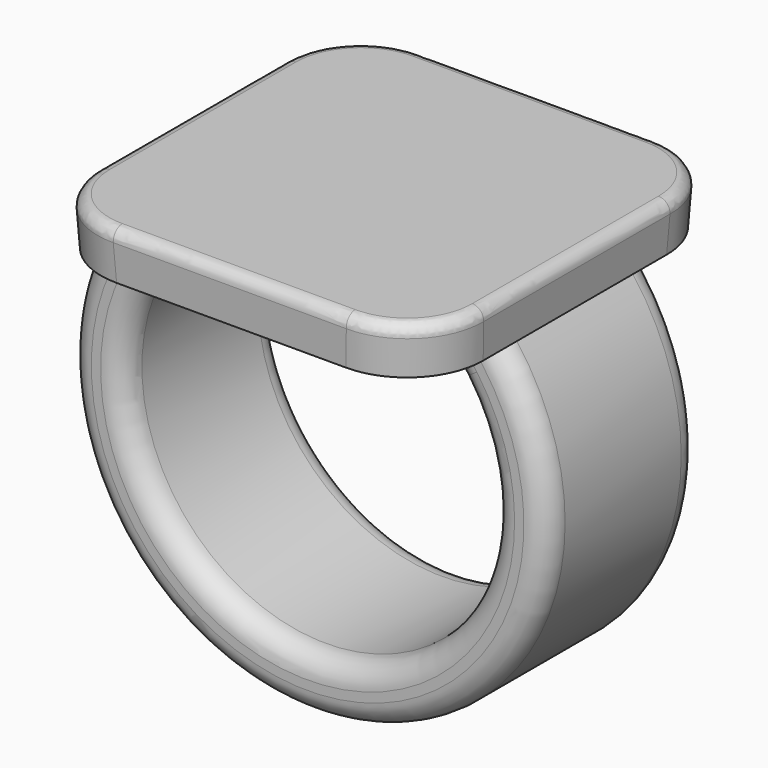
from build123d import *

# Parameters (mm, degrees)
F0_W          = 25.4
F0_H          = 25.4
F1_DEPTH      = 3.175
F1_TAPER      = -3
F3_W          = 5.08
F3_H          = 12.7
F6_DEPTH      = 6.35
F6_DEPTH_BACK = 6.35
F7_R          = 5.08
F8_R          = 1.524
F9_R          = 0.762


# Not quite as in the source:
# - a feature names something its author has since deleted; it is built from what else it names


with BuildPart() as f1:
    # F0 (on Top) → F1 (new body)
    with BuildSketch(Plane.XY):
        Rectangle(F0_W, F0_H)
    extrude(amount=F1_DEPTH, taper=F1_TAPER)

    # F4: sweep along a path in F2
    with BuildLine(Plane.XZ) as f4_path:
        ThreePointArc((-10.16, 0), (0, -23.5582897328), (10.16, 0))
    # F3 (on face) → F4 (sweep)
    with BuildSketch(Plane(origin=(0, 0, 0), x_dir=(1, 0, 0), z_dir=(0, 0, -1))):
        with Locations((-10.16, 0)):
            Rectangle(F3_W, F3_H)
    sweep(path=f4_path.line)

    # F5 (on Front) → F6 (join, two sides)
    with BuildSketch(Plane.XZ) as f6_sk:
        with BuildLine():
            Line((10.0130578512, -2.535746045), (10.16, 0))
            Line((10.16, 0), (7.62, 0))
            ThreePointArc((7.62, 0), (8.9072265211, -1.1822790439), (10.0130578512, -2.535746045))
        make_face()
    extrude(amount=F6_DEPTH)
    extrude(f6_sk.sketch, amount=-F6_DEPTH_BACK)

    # F7
    f7_edges = [f1.edges().sort_by_distance(p)[0] for p in [
        (-12.783197, 12.783197, 1.5875),
        (-12.783197, -12.783197, 1.5875),
        (12.783197, -12.783197, 1.5875),
        (12.783197, 12.783197, 1.5875),
    ]]
    fillet(f7_edges, radius=F7_R)

    # F8
    f8_edges = [f1.edges().sort_by_distance(p)[0] for p in [
        (-1.743325, -6.35, -21.711017),
        (8.907227, -6.35, -1.182279),
        (-1.743325, 6.35, -21.711017),
        (0, -6.35, -25.501344),
        (8.907227, 6.35, -1.182279),
        (0, 6.35, -25.501344),
    ]]
    fillet(f8_edges, radius=F8_R)

    # F9
    f9_edges = [f1.edges().sort_by_distance(p)[0] for p in [
        (0, -12.866395, 3.175),
        (-11.381378, -11.381378, 3.175),
        (11.381378, -11.381378, 3.175),
        (-12.866395, 0, 3.175),
        (12.866395, 0, 3.175),
        (-11.381378, 11.381378, 3.175),
        (11.381378, 11.381378, 3.175),
        (0, 12.866395, 3.175),
    ]]
    fillet(f9_edges, radius=F9_R)


solid = f1.part
